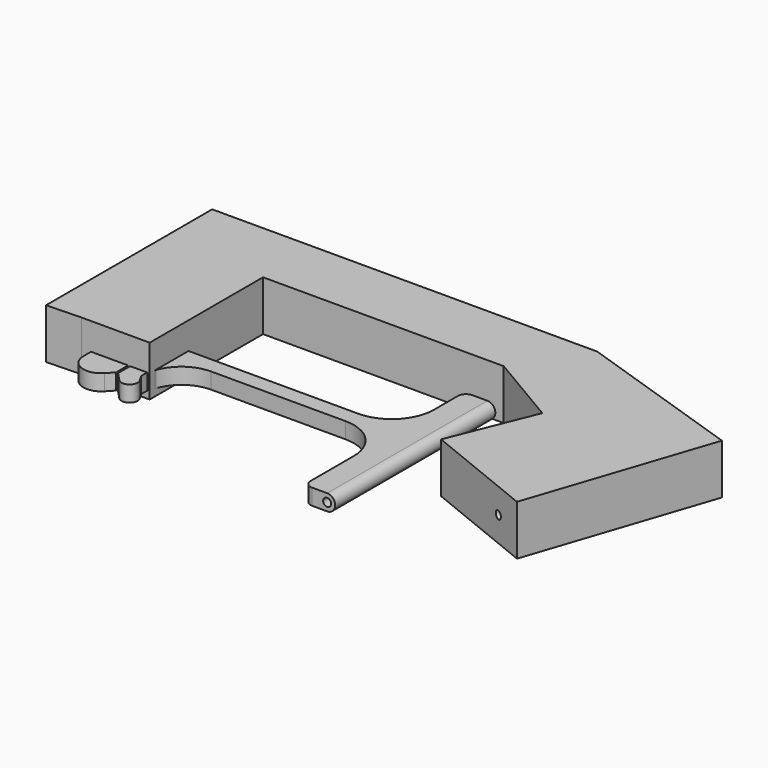
from build123d import *

# Parameters (mm, degrees)
F3_DEPTH  = 25
F4_R      = 2
F5_REACH  = 179.0646776001
F7_DEPTH  = 15
F8_R      = 2
F9_DEPTH  = 100.001
F10_W     = 4
F10_H     = 3.5
F10_W_2   = 21
F10_W_3   = 100
F10_W_4   = 14
F11_DEPTH = 100.001


# Not quite as in the source:
# - the program builds the solid bodies; features that only make, move or delete a surface that nothing else refers to are left out


with BuildPart() as f3:
    # F2 (on Top) → F3 (new body)
    with BuildSketch(Plane.XY):
        Polygon((-41.0616472363, -7.7508748509), (-23.7303264439, -7.237566635), (10.2535411716, -7.237566635), (10.2535411716, 63.5198950768), (130.4651498795, 63.5198950768), (166.9851094484, 41.9629588723), (149.9931961298, 0), (206.0509233637, -22.6992582886), (236.1825853586, 67.5677359104), (151.1922137485, 95.9380297581), (-41.0616472363, 95.9380297581), align=None)
    extrude(amount=F3_DEPTH)

    f5_end = f3.faces().sort_by_distance((178.0220597468, -11.3496291443, 12.5))[0]
    # F4 (on face) → F5 (cut, up to a face of the model that its end follows)
    with BuildSketch(Plane(origin=(43.9718677966, 131.7288218617, 0), x_dir=(-0.9485487152, 0.3166312286, 0), z_dir=(0.3166312286, 0.9485487152, 0))):
        with Locations((-187.8149360418, 12.5)):
            Circle(F4_R)
    f5_long = extrude(amount=-F5_REACH, mode=Mode.PRIVATE)
    add(split(f5_long, bisect_by=f5_end, keep=Keep.BOTTOM, mode=Mode.PRIVATE), mode=Mode.SUBTRACT)


with BuildPart() as f7:
    # F6 (on Top) → F7 (new body)
    with BuildSketch(Plane.XY):
        with BuildLine():
            ThreePointArc((108.5646599662, 17), (106.9006209041, 16.0142040831), (105.1653529206, 15.16))
            ThreePointArc((105.1653529206, 15.16), (118.8306025385, 4.5258095914), (124, -12))
            Line((124, -12), (124, -39))
            ThreePointArc((124, -39), (122.8284271247, -41.8284271247), (120, -43))
            Line((120, -43), (135, -43))
            Line((135, -43), (135, 17))
            Line((135, 17), (124, 17))
            Line((124, 17), (108.5646599662, 17))
        make_face()
        with BuildLine():
            Line((-0.5, -7.7916666667), (-2.8378378378, -0.972972973))
            ThreePointArc((-2.8378378378, -0.972972973), (0, 3), (2.8378378378, -0.972972973))
            Line((2.8378378378, -0.972972973), (0.5, -7.7916666667))
            Line((0.5, -7.7916666667), (0.5, -14.7755569556))
            Line((0.5, -14.7755569556), (4.6019879687, -19.087213573))
            ThreePointArc((4.6019879687, -19.087213573), (9.8953251293, -19.5336278423), (10.9641016151, -14.3301270189))
            Line((10.9641016151, -14.3301270189), (9, -10.9282032303))
            Line((9, -10.9282032303), (9, -7.6666666667))
            Line((9, -7.6666666667), (10.4054054054, -3.5675675676))
            ThreePointArc((10.4054054054, -3.5675675676), (17.1889695968, 5.5354425644), (28, 9))
            Line((28, 9), (95, 9))
            ThreePointArc((95, 9), (109.8492424049, 2.8492424049), (116, -12))
            Line((116, -12), (116, -39))
            ThreePointArc((116, -39), (117.1715728753, -41.8284271247), (120, -43))
            ThreePointArc((120, -43), (122.8284271247, -41.8284271247), (124, -39))
            Line((124, -39), (124, -12))
            ThreePointArc((124, -12), (118.8306025385, 4.5258095914), (105.1653529206, 15.16))
            ThreePointArc((105.1653529206, 15.16), (100.1652686281, 16.5362926814), (95, 17))
            Line((95, 17), (-5, 17))
            ThreePointArc((-5, 17), (-14.8994949366, 12.8994949366), (-19, 3))
            Line((-19, 3), (-19, -12))
            ThreePointArc((-19, -12), (-13.4147336478, -20.247270588), (-3.6835816648, -18.1218639308))
            Line((-3.6835816648, -18.1218639308), (-0.5, -14.7755569556))
            Line((-0.5, -14.7755569556), (-0.5, -7.7916666667))
        make_face()
        with BuildLine():
            ThreePointArc((116, 38), (109.8492424049, 23.1507575951), (95, 17))
            Line((95, 17), (108.5646599662, 17))
            Line((108.5646599662, 17), (124, 17))
            Line((124, 17), (135, 17))
            Line((135, 17), (135, 57))
            Line((135, 57), (120, 57))
            ThreePointArc((120, 57), (117.1715728753, 55.8284271247), (116, 53))
            Line((116, 53), (116, 38))
        make_face()
        with BuildLine():
            Line((108.5646599662, 17), (95, 17))
            ThreePointArc((95, 17), (100.1652686281, 16.5362926814), (105.1653529206, 15.16))
            ThreePointArc((105.1653529206, 15.16), (106.9006209041, 16.0142040831), (108.5646599662, 17))
        make_face()
    extrude(amount=F7_DEPTH)

    # F8 (on face) → F9 (cut, through all)
    with BuildSketch(Plane(origin=(0, 57, 0), x_dir=(-1, 0, 0), z_dir=(0, 1, 0))):
        with Locations((-127.5, 7.5)):
            Circle(F8_R)
    extrude(amount=-F9_DEPTH, mode=Mode.SUBTRACT)

    # F10 (on face) → F11 (cut, through all)
    with BuildSketch(Plane(origin=(0, 57, 0), x_dir=(-1, 0, 0), z_dir=(0, 1, 0))):
        with BuildLine():
            ThreePointArc((-127.5, 3.5), (-131.5, 7.5), (-127.5, 11.5))
            Line((-127.5, 11.5), (-120, 11.5))
            Line((-120, 11.5), (-120, 15))
            Line((-120, 15), (-135, 15))
            Line((-135, 15), (-135, 0))
            Line((-135, 0), (-120, 0))
            Line((-120, 0), (-120, 3.5))
            Line((-120, 3.5), (-127.5, 3.5))
        make_face()
        with Locations((-118, 13.25)):
            Rectangle(F10_W, F10_H)
        with Locations((-105.5, 13.25)):
            Rectangle(F10_W_2, F10_H)
        with Locations((-118, 1.75)):
            Rectangle(F10_W, F10_H)
        with Locations((-105.5, 1.75)):
            Rectangle(F10_W_2, F10_H)
        with Locations((-45, 1.75)):
            Rectangle(F10_W_3, F10_H)
        with Locations((-45, 13.25)):
            Rectangle(F10_W_3, F10_H)
        with Locations((12, 13.25)):
            Rectangle(F10_W_4, F10_H)
        with Locations((12, 1.75)):
            Rectangle(F10_W_4, F10_H)
    extrude(amount=-F11_DEPTH, mode=Mode.SUBTRACT)


solid = Compound([f3.part, f7.part])
